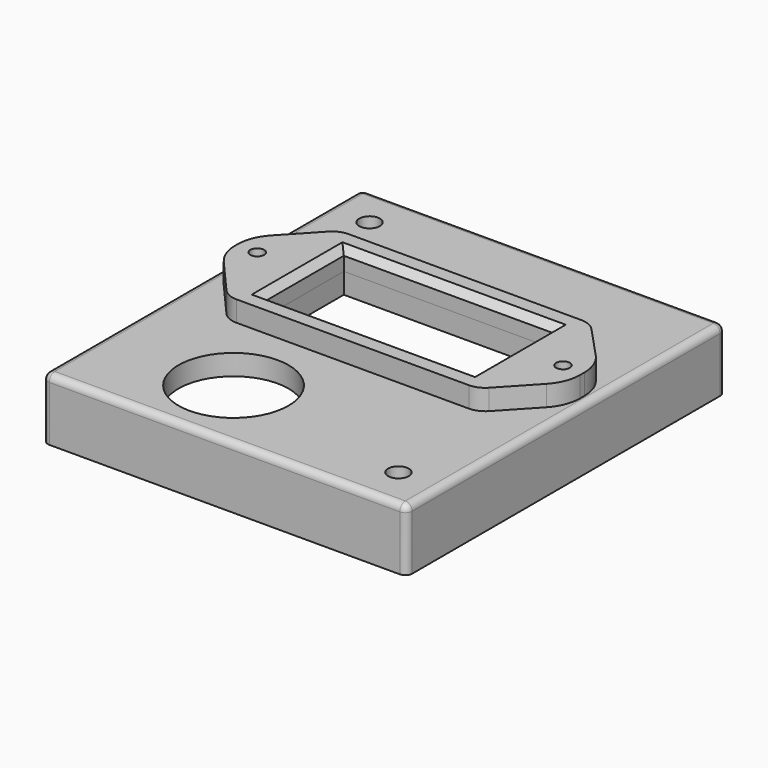
from build123d import *

# Parameters (mm, degrees)
F0_W      = 51
F0_H      = 56
F0_R      = 6.1
F0_R_2    = 1.5
F0_W_2    = 5
F0_H_2    = 14.5
F1_DEPTH  = 1
F2_W      = 30
F2_H      = 14
F5_DEPTH  = 4
F2_W_2    = 51
F2_H_2    = 56
F2_R      = 8
F2_R_2    = 1.5
F2_R_3    = 0.8
F2_W_3    = 30.5
F2_H_3    = 14.5
F6_DEPTH  = 3
F2_W_4    = 5
F2_H_4    = 2
F2_H_5    = 5
F7_DEPTH  = 2
F3_W      = 27.8
F3_H      = 11.8
F8_DEPTH  = 1.5
F2_H_6    = 1
F9_DEPTH  = 9
F10_W     = 36.5
F10_H     = 20.5
F10_W_2   = 30.5
F10_H_2   = 14.5
F10_R     = 1
F11_DEPTH = 3
F12_R     = 6
F13_R     = 3
F14_R     = 1
F15_SIZE  = 1
F18_DEPTH = 1
F19_D     = 1.4
F19_DEPTH = 1.001
F21_D     = 1.4
F16_W     = 51
F16_H     = 56
F16_W_2   = 25
F16_H_2   = 18
F16_R     = 1.5
F22_DEPTH = 5
F23_W     = 0.2
F23_H     = 55.6
F24_DEPTH = 25
F25_D     = 1.6
F25_DEPTH = 5.001
F26_D     = 1.6


# Not quite as in the source:
# - a feature names something its author has since deleted; it is built from what else it names


with BuildPart() as f1:
    # F0 (on Top) → F1 (new body)
    with BuildSketch(Plane.XY):
        Rectangle(F0_W, F0_H)
        with Locations((-7.5, -18)):
            Circle(F0_R, mode=Mode.SUBTRACT)
        with Locations((20.5, -23)):
            Circle(F0_R_2, mode=Mode.SUBTRACT)
        with Locations((-20.5, 23)):
            Circle(F0_R_2, mode=Mode.SUBTRACT)
        Polygon((-15.25, -2.75), (-15.25, 11.75), (-2.5, 11.75), (2.5, 11.75), (15.25, 11.75), (15.25, -2.75), (2.5, -2.75), (-2.5, -2.75), align=None, mode=Mode.SUBTRACT)
        with Locations((0, 4.5)):
            Rectangle(F0_W_2, F0_H_2)
    extrude(amount=F1_DEPTH)

    # F18 (add): a face of the model
    f18_faces = [f1.faces().sort_by_distance(p)[0] for p in [
        (0.3722548806, 0.1869472989, 1),
    ]]
    extrude(f18_faces, amount=F18_DEPTH)

    # F19 (through all, one way)
    with BuildSketch(Plane.XY.offset(1)):
        with Locations((-22.25, 4.75), (22.25, 4.75)):
            Circle(F19_D / 2)
    extrude(amount=-F19_DEPTH, mode=Mode.SUBTRACT)

    # F21 (through all)
    with Locations(Plane(origin=(0, 0, 1), x_dir=(1, 0, 0), z_dir=(0, 0, -1))):
        with Locations((-22.25, -4.75), (22.25, -4.75)):
            Hole(F21_D / 2)

    # F16 (on face) → F22 (join)
    with BuildSketch(Plane.XY.offset(1)):
        Rectangle(F16_W, F16_H)
        with Locations((-7.5, -18)):
            Rectangle(F16_W_2, F16_H_2, mode=Mode.SUBTRACT)
        with Locations((20.5, -23)):
            Circle(F16_R, mode=Mode.SUBTRACT)
        with Locations((-20.5, 23)):
            Circle(F16_R, mode=Mode.SUBTRACT)
        Polygon((-15.25, -2.75), (-15.25, 11.75), (-2.5, 11.75), (2.5, 11.75), (15.25, 11.75), (15.25, -2.75), (2.5, -2.75), (-2.5, -2.75), align=None, mode=Mode.SUBTRACT)
    extrude(amount=F22_DEPTH)

    # F23 (on face) → F24 (cut)
    with BuildSketch(Plane(origin=(0, 0, 0), x_dir=(1, 0, 0), z_dir=(0, 0, -1))):
        Polygon((25.5, 28), (-25.5, 28), (-25.5, 27.8), (-25.3, 27.8), (25.3, 27.8), (25.5, 27.8), align=None)
        with Locations((-25.4, 0)):
            Rectangle(F23_W, F23_H)
        with Locations((25.4, 0)):
            Rectangle(F23_W, F23_H)
        Polygon((-25.3, -27.8), (-25.5, -27.8), (-25.5, -28), (25.5, -28), (25.5, -27.8), (25.3, -27.8), align=None)
    extrude(amount=-F24_DEPTH, mode=Mode.SUBTRACT)

    # F25 (through all, one way)
    with BuildSketch(Plane(origin=(0, 0, 1), x_dir=(1, 0, 0), z_dir=(0, 0, -1))):
        with Locations((-22.25, -4.75), (22.25, -4.75)):
            Circle(F25_D / 2)
    extrude(amount=-F25_DEPTH, mode=Mode.SUBTRACT)

    # F26 (through all)
    with Locations(Plane.XY.offset(1)):
        with Locations((22.25, 4.75), (-22.25, 4.75)):
            Hole(F26_D / 2)


with BuildPart() as f5:
    # F2 (on Top) → F5 (new body)
    with BuildSketch(Plane.XY):
        with Locations((-48.0005137329, -108.0776734079)):
            Rectangle(F2_W, F2_H)
        Polygon((-62.0005137329, -114.0776734079), (-62.0005137329, -102.0776734079), (-50.5005137329, -102.0776734079), (-45.5005137329, -102.0776734079), (-34.0005137329, -102.0776734079), (-34.0005137329, -107.0776734079), (-34.0005137329, -109.0776734079), (-34.0005137329, -114.0776734079), (-45.5005137329, -114.0776734079), (-50.5005137329, -114.0776734079), align=None, mode=Mode.SUBTRACT)
    extrude(amount=F5_DEPTH)

    # F2 (on Top) → F7 (join)
    with BuildSketch(Plane.XY):
        with Locations((-48.0005137329, -108.0776734079)):
            Rectangle(F2_W_4, F2_H_4)
        with Locations((-48.0005137329, -104.5776734079)):
            Rectangle(F2_W_4, F2_H_5)
        with Locations((-48.0005137329, -111.5776734079)):
            Rectangle(F2_W_4, F2_H_5)
    extrude(amount=F7_DEPTH)


with BuildPart() as f6:
    # F2 (on Top) → F6 (new body)
    with BuildSketch(Plane.XY):
        with Locations((28.2103444552, -118.9687541723)):
            Rectangle(F2_W_2, F2_H_2)
        with Locations((20.7103444552, -136.9687541723)):
            Circle(F2_R, mode=Mode.SUBTRACT)
        with Locations((48.7103444552, -141.9687541723)):
            Circle(F2_R_2, mode=Mode.SUBTRACT)
        with Locations((5.9603444552, -114.2187541723)):
            Circle(F2_R_3, mode=Mode.SUBTRACT)
        with Locations((28.2103444552, -114.4687541723)):
            Rectangle(F2_W_3, F2_H_3, mode=Mode.SUBTRACT)
        with Locations((50.4603444552, -114.2187541723)):
            Circle(F2_R_3, mode=Mode.SUBTRACT)
        with Locations((7.7103444552, -95.9687541723)):
            Circle(F2_R_2, mode=Mode.SUBTRACT)
    extrude(amount=-F6_DEPTH)

    # F2 (on Top) → F9 (join)
    with BuildSketch(Plane.XY):
        Polygon((2.7103444552, -146.9687541723), (2.7103444552, -90.9687541723), (2.7103444552, -89.9687541723), (1.7103444552, -89.9687541723), (1.7103444552, -147.9687541723), (2.7103444552, -147.9687541723), align=None)
        with Locations((28.2103444552, -90.4687541723)):
            Rectangle(F2_W_2, F2_H_6)
        with Locations((28.2103444552, -147.4687541723)):
            Rectangle(F2_W_2, F2_H_6)
        Polygon((53.7103444552, -89.9687541723), (53.7103444552, -90.9687541723), (53.7103444552, -146.9687541723), (53.7103444552, -147.9687541723), (54.7103444552, -147.9687541723), (54.7103444552, -89.9687541723), align=None)
    extrude(amount=-F9_DEPTH)

    # F14
    f14_edges = [f6.edges().sort_by_distance(p)[0] for p in [
        (1.710344, -118.968754, 0),
        (28.210344, -89.968754, 0),
        (28.210344, -147.968754, 0),
        (54.710344, -118.968754, 0),
        (54.710344, -147.968754, -4.5),
        (1.710344, -147.968754, -4.5),
        (1.710344, -89.968754, -4.5),
        (54.710344, -89.968754, -4.5),
    ]]
    fillet(f14_edges, radius=F14_R)


with BuildPart() as f8:
    # F3 (on Top) → F8 (new body)
    with BuildSketch(Plane.XY):
        with Locations((-52.0366017878, -79.3675661445)):
            Rectangle(F3_W, F3_H)
    extrude(amount=F8_DEPTH)


with BuildPart() as f11:
    # F10 (on face) → F11 (new body)
    with BuildSketch(Plane.XY):
        with Locations((28.2103444552, -114.4687541723)):
            Rectangle(F10_W, F10_H)
        with Locations((28.2103444552, -114.4687541723)):
            Rectangle(F10_W_2, F10_H_2, mode=Mode.SUBTRACT)
        Polygon((9.9603444552, -124.7187541723), (9.9603444552, -104.2187541723), (2.9603444552, -111.7187541723), (2.9603444552, -116.7187541723), align=None)
        with Locations((5.9603444552, -114.2187541723)):
            Circle(F10_R, mode=Mode.SUBTRACT)
        Polygon((53.4603444552, -111.7187541723), (46.4603444552, -104.2187541723), (46.4603444552, -124.7187541723), (53.4603444552, -117.2187541723), align=None)
        with Locations((50.4603444552, -114.2187541723)):
            Circle(F10_R, mode=Mode.SUBTRACT)
    extrude(amount=F11_DEPTH)

    # F12
    f12_edges = [f11.edges().sort_by_distance(p)[0] for p in [
        (2.960344, -111.718754, 1.5),
        (2.960344, -116.718754, 1.5),
        (53.460344, -117.218754, 1.5),
        (53.460344, -111.718754, 1.5),
    ]]
    fillet(f12_edges, radius=F12_R)

    # F13
    f13_edges = [f11.edges().sort_by_distance(p)[0] for p in [
        (9.960344, -104.218754, 1.5),
        (9.960344, -124.718754, 1.5),
        (46.460344, -124.718754, 1.5),
        (46.460344, -104.218754, 1.5),
    ]]
    fillet(f13_edges, radius=F13_R)

    # F15
    f15_edges = [f11.edges().sort_by_distance(p)[0] for p in [
        (12.960344, -114.468754, 3),
        (28.210344, -107.218754, 3),
        (43.460344, -114.468754, 3),
        (28.210344, -121.718754, 3),
    ]]
    chamfer(f15_edges, length=F15_SIZE)


solid = Compound([f6.part, f11.part])
